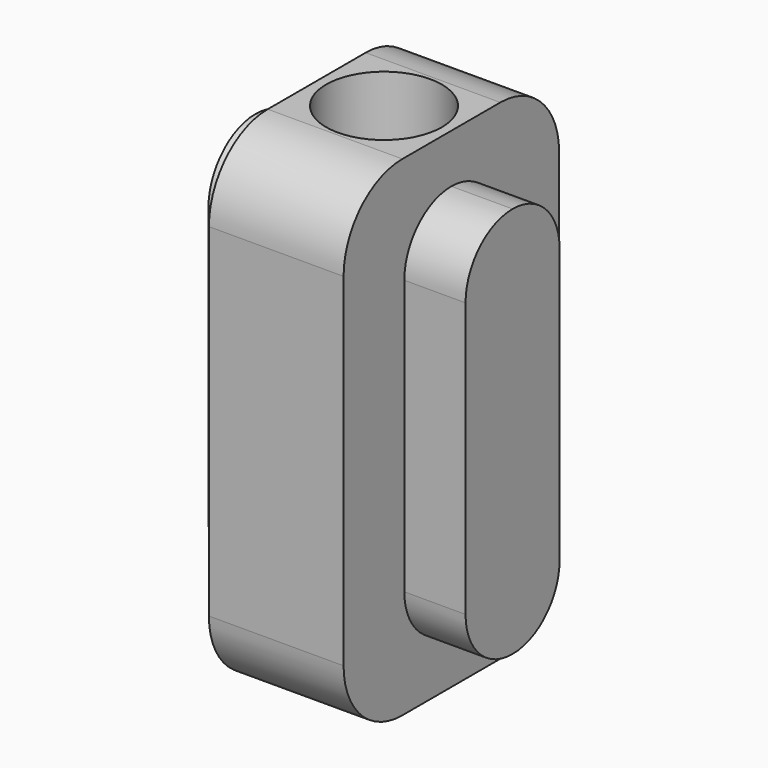
from build123d import *

# Parameters (mm, degrees)
F0_W     = 6.985
F0_H     = 13.97
F1_DEPTH = 25.4
F2_R     = 3
F3_DEPTH = 25.4
F4_W     = 3.048
F4_H     = 20.32
F5_DEPTH = 3.175
F6_R     = 3.04799
F8_R     = 3.81


# Not quite as in the source:
# - a fillet or chamfer is up to 0.001 mm smaller than in the source, because OpenCascade refuses the exact size


with BuildPart() as f1:
    # F0 (on Top) → F1 (new body)
    with BuildSketch(Plane.XY):
        Rectangle(F0_W, F0_H)
    extrude(amount=F1_DEPTH)

    # F2 (on face) → F3 (cut)
    with BuildSketch(Plane(origin=(0, 0, 0), x_dir=(1, 0, 0), z_dir=(0, 0, -1))):
        Circle(F2_R)
    extrude(amount=-F3_DEPTH, mode=Mode.SUBTRACT)

    # F4 (on face) → F5 (join)
    with BuildSketch(Plane.YZ.offset(3.4925)):
        with Locations((1.524, 12.7)):
            Rectangle(F4_W, F4_H)
        with Locations((-1.524, 12.7)):
            Rectangle(F4_W, F4_H)
    extrude(amount=F5_DEPTH)

    # F6 (radius 3.048 in the source; OpenCascade refuses exactly that, so slightly less here)
    f6_edges = [f1.edges().sort_by_distance(p)[0] for p in [
        (5.08, -3.048, 22.86),
        (5.08, 3.048, 22.86),
        (5.08, 3.048, 2.54),
        (5.08, -3.048, 2.54),
    ]]
    fillet(f6_edges, radius=F6_R)

    # F7: F1 across plane


with BuildPart() as f1_1:
    add(f1.part)
    add(f1.part.mirror(Plane.YZ))

    # F8
    f8_edges = [f1_1.edges().sort_by_distance(p)[0] for p in [
        (0, -6.985, 0),
        (0, 6.985, 0),
        (0, 6.985, 25.4),
        (0, -6.985, 25.4),
    ]]
    fillet(f8_edges, radius=F8_R)


solid = f1_1.part
